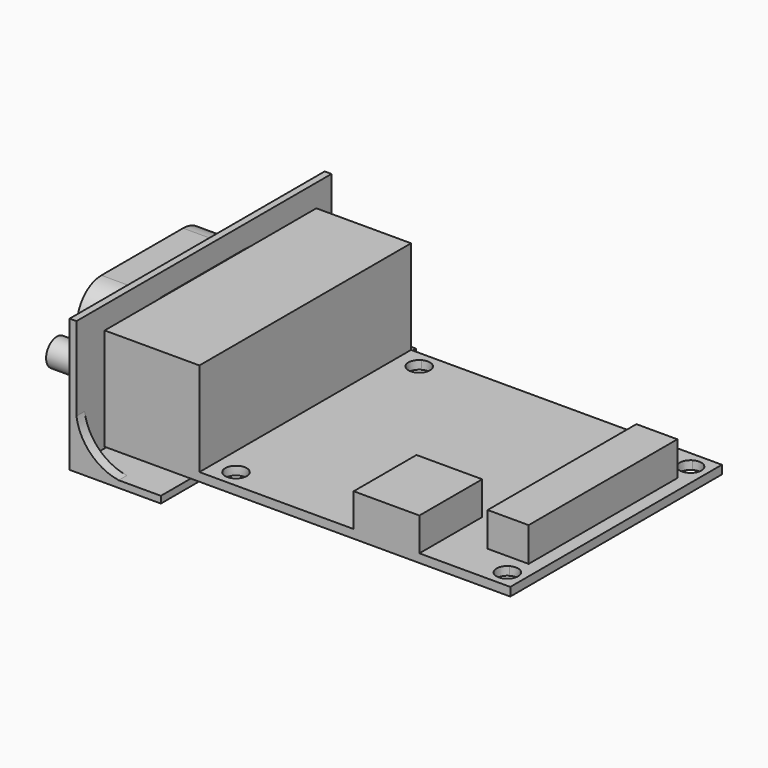
from build123d import *

# Parameters (mm, degrees)
F0_W           = 47.5266514695
F0_H           = 31
F1_DEPTH       = 1
F2_W           = 4.8044053313
F2_H           = 21.7868040781
F3_DEPTH       = 5
F4_W           = 11.1009664834
F4_H           = 31
F5_DEPTH       = 12
F7_R           = 1.5875
F8_DEPTH       = 8
F9_W           = 7.7
F9_H           = 9.2
F10_DEPTH      = 4.9
F11_W          = 55
F11_H          = 37.359307176
F12_DEPTH      = 14
F12_DEPTH_BACK = 1.6
F13_T          = -0.8
F14_OFFSET     = 0.2
F15_W          = 48.7006613985
F15_H          = 51.2911211699
F16_DEPTH      = 25
F18_DEPTH      = 1.2


# Not quite as in the source:
# - ends of sketch curves that miss each other by under 0.0002 mm in the source are joined
# - a pattern or mirror of a feature is missing from the dataset's text; its kind, count and spacing are read off the source's solid


with BuildPart() as f1:
    # F0 (on Top) → F1 (new body)
    with BuildSketch(Plane.XY):
        with Locations((1.27e-05, -1.27e-05)):
            Rectangle(F0_W, F0_H)
        with BuildLine():
            add(Edge.make_bspline(
                [(-13.943801891, -11.7896289619), (-13.943801891, -11.298779652), (-14.205665174, -10.8452147748), (-14.6307564405, -10.5997901198)],
                knots=[0, 0, 0, 0, 1, 1, 1, 1], degree=3))
            add(Edge.make_bspline(
                [(-14.6307564405, -12.9794642726), (-14.205665174, -12.7340396176), (-13.943801891, -12.2804782718), (-13.943801891, -11.7896289619)],
                knots=[0, 0, 0, 0, 1, 1, 1, 1], degree=3))
            add(Edge.make_bspline(
                [(-16.0046620081, -12.9794642726), (-15.5795707416, -13.2248889276), (-15.0558441757, -13.2248889276), (-14.6307564405, -12.9794642726)],
                knots=[0, 0, 0, 0, 1, 1, 1, 1], degree=3))
            add(Edge.make_bspline(
                [(-16.6916130263, -11.7896289619), (-16.6916130263, -12.2804782718), (-16.4297497433, -12.7340396176), (-16.0046620081, -12.9794642726)],
                knots=[0, 0, 0, 0, 1, 1, 1, 1], degree=3))
            add(Edge.make_bspline(
                [(-16.0046620081, -10.5997901198), (-16.4297497433, -10.8452147748), (-16.6916130263, -11.298779652), (-16.6916130263, -11.7896289619)],
                knots=[0, 0, 0, 0, 1, 1, 1, 1], degree=3))
            add(Edge.make_bspline(
                [(-14.6307564405, -10.5997901198), (-15.0558441757, -10.3543654648), (-15.5795707416, -10.3543654648), (-16.0046620081, -10.5997901198)],
                knots=[0, 0, 0, 0, 1, 1, 1, 1], degree=3))
        make_face(mode=Mode.SUBTRACT)
        with BuildLine():
            add(Edge.make_bspline(
                [(-8.7818043126, -13.417529872), (-8.7818043126, -12.7211853521), (-9.3463043262, -12.1566853385), (-10.0426488461, -12.1566853385)],
                knots=[0, 0, 0, 0, 1, 1, 1, 1], degree=3))
            add(Edge.make_bspline(
                [(-9.4122248137, -14.5094538185), (-9.0221190439, -14.2842287237), (-8.7818043126, -13.8679871245), (-8.7818043126, -13.417529872)],
                knots=[0, 0, 0, 0, 1, 1, 1, 1], degree=3))
            add(Edge.make_bspline(
                [(-10.6730728785, -14.5094538185), (-10.2829635774, -14.7346824448), (-9.8023341148, -14.7346824448), (-9.4122248137, -14.5094538185)],
                knots=[0, 0, 0, 0, 1, 1, 1, 1], degree=3))
            add(Edge.make_bspline(
                [(-11.3034933795, -13.417529872), (-11.3034933795, -13.8679871245), (-11.0631786482, -14.2842287237), (-10.6730728785, -14.5094538185)],
                knots=[0, 0, 0, 0, 1, 1, 1, 1], degree=3))
            add(Edge.make_bspline(
                [(-10.0426488461, -12.1566853385), (-10.7389933659, -12.1566853385), (-11.3034933795, -12.7211853521), (-11.3034933795, -13.417529872)],
                knots=[0, 0, 0, 0, 1, 1, 1, 1], degree=3))
        make_face(mode=Mode.SUBTRACT)
        with BuildLine():
            add(Edge.make_bspline(
                [(23.0153119985, -13.4241830138), (23.0153119985, -12.9737257612), (22.7749937359, -12.5574841621), (22.3848879661, -12.3322555358)],
                knots=[0, 0, 0, 0, 1, 1, 1, 1], degree=3))
            add(Edge.make_bspline(
                [(22.3848879661, -14.5161069604), (22.7749937359, -14.2908783341), (23.0153119985, -13.8746367349), (23.0153119985, -13.4241830138)],
                knots=[0, 0, 0, 0, 1, 1, 1, 1], degree=3))
            add(Edge.make_bspline(
                [(21.1240434327, -14.5161069604), (21.5141492024, -14.7413355866), (21.9947821964, -14.7413355866), (22.3848879661, -14.5161069604)],
                knots=[0, 0, 0, 0, 1, 1, 1, 1], degree=3))
            add(Edge.make_bspline(
                [(20.4936194003, -13.4241830138), (20.4936194003, -13.8746367349), (20.7339341315, -14.2908783341), (21.1240434327, -14.5161069604)],
                knots=[0, 0, 0, 0, 1, 1, 1, 1], degree=3))
            add(Edge.make_bspline(
                [(21.1240434327, -12.3322555358), (20.7339341315, -12.5574841621), (20.4936194003, -12.9737257612), (20.4936194003, -13.4241830138)],
                knots=[0, 0, 0, 0, 1, 1, 1, 1], degree=3))
            add(Edge.make_bspline(
                [(22.3848879661, -12.3322555358), (21.9947821964, -12.1070304409), (21.5141492024, -12.1070304409), (21.1240434327, -12.3322555358)],
                knots=[0, 0, 0, 0, 1, 1, 1, 1], degree=3))
        make_face(mode=Mode.SUBTRACT)
        with BuildLine():
            add(Edge.make_bspline(
                [(-14.6307564405, 12.9794353412), (-14.205665174, 12.7340106862), (-13.943801891, 12.2804493404), (-13.943801891, 11.7896000305)],
                knots=[0, 0, 0, 0, 1, 1, 1, 1], degree=3))
            add(Edge.make_bspline(
                [(-13.943801891, 11.7896000305), (-13.943801891, 11.2987507206), (-14.205665174, 10.8451858434), (-14.6307564405, 10.5997611884)],
                knots=[0, 0, 0, 0, 1, 1, 1, 1], degree=3))
            add(Edge.make_bspline(
                [(-14.6307564405, 10.5997611884), (-15.0558441757, 10.3543365334), (-15.5795707416, 10.3543365334), (-16.0046620081, 10.5997611884)],
                knots=[0, 0, 0, 0, 1, 1, 1, 1], degree=3))
            add(Edge.make_bspline(
                [(-16.0046620081, 10.5997611884), (-16.4297497433, 10.8451858434), (-16.6916130263, 11.2987507206), (-16.6916130263, 11.7896000305)],
                knots=[0, 0, 0, 0, 1, 1, 1, 1], degree=3))
            add(Edge.make_bspline(
                [(-16.6916130263, 11.7896000305), (-16.6916130263, 12.2804493404), (-16.4297497433, 12.7340106862), (-16.0046620081, 12.9794353412)],
                knots=[0, 0, 0, 0, 1, 1, 1, 1], degree=3))
            add(Edge.make_bspline(
                [(-16.0046620081, 12.9794353412), (-15.5795707416, 13.2248599962), (-15.0558441757, 13.2248599962), (-14.6307564405, 12.9794353412)],
                knots=[0, 0, 0, 0, 1, 1, 1, 1], degree=3))
        make_face(mode=Mode.SUBTRACT)
        with BuildLine():
            add(Edge.make_bspline(
                [(-9.4122248137, 14.5094248872), (-9.0221190439, 14.2841962609), (-8.7818043126, 13.8679581931), (-8.7818043126, 13.4175009406)],
                knots=[0, 0, 0, 0, 1, 1, 1, 1], degree=3))
            add(Edge.make_bspline(
                [(-8.7818043126, 13.4175009406), (-8.7818043126, 12.7211564207), (-9.3463043262, 12.1566564071), (-10.0426488461, 12.1566564071)],
                knots=[0, 0, 0, 0, 1, 1, 1, 1], degree=3))
            add(Edge.make_bspline(
                [(-10.0426488461, 12.1566564071), (-10.7389933659, 12.1566564071), (-11.3034933795, 12.7211564207), (-11.3034933795, 13.4175009406)],
                knots=[0, 0, 0, 0, 1, 1, 1, 1], degree=3))
            add(Edge.make_bspline(
                [(-11.3034933795, 13.4175009406), (-11.3034933795, 13.8679581931), (-11.0631786482, 14.2841962609), (-10.6730728785, 14.5094248872)],
                knots=[0, 0, 0, 0, 1, 1, 1, 1], degree=3))
            add(Edge.make_bspline(
                [(-10.6730728785, 14.5094248872), (-10.2829635774, 14.7346535134), (-9.8023341148, 14.7346535134), (-9.4122248137, 14.5094248872)],
                knots=[0, 0, 0, 0, 1, 1, 1, 1], degree=3))
        make_face(mode=Mode.SUBTRACT)
        with BuildLine():
            add(Edge.make_bspline(
                [(22.3848879661, 14.516078029), (22.7749937359, 14.2908494027), (23.0153119985, 13.8746078036), (23.0153119985, 13.424150551)],
                knots=[0, 0, 0, 0, 1, 1, 1, 1], degree=3))
            add(Edge.make_bspline(
                [(23.0153119985, 13.424150551), (23.0153119985, 12.9736968298), (22.7749937359, 12.5574552307), (22.3848879661, 12.3322266044)],
                knots=[0, 0, 0, 0, 1, 1, 1, 1], degree=3))
            add(Edge.make_bspline(
                [(22.3848879661, 12.3322266044), (21.9947821964, 12.1069979781), (21.5141492024, 12.1069979781), (21.1240434327, 12.3322266044)],
                knots=[0, 0, 0, 0, 1, 1, 1, 1], degree=3))
            add(Edge.make_bspline(
                [(21.1240434327, 12.3322266044), (20.7339341315, 12.5574552307), (20.4936194003, 12.9736968298), (20.4936194003, 13.424150551)],
                knots=[0, 0, 0, 0, 1, 1, 1, 1], degree=3))
            add(Edge.make_bspline(
                [(20.4936194003, 13.424150551), (20.4936194003, 13.8746078036), (20.7339341315, 14.2908494027), (21.1240434327, 14.516078029)],
                knots=[0, 0, 0, 0, 1, 1, 1, 1], degree=3))
            add(Edge.make_bspline(
                [(21.1240434327, 14.516078029), (21.5141492024, 14.7413066552), (21.9947821964, 14.7413066552), (22.3848879661, 14.516078029)],
                knots=[0, 0, 0, 0, 1, 1, 1, 1], degree=3))
        make_face(mode=Mode.SUBTRACT)
    extrude(amount=F1_DEPTH)

    # F2 (on Top) → F3 (join)
    with BuildSketch(Plane.XY):
        with Locations((19.8277348989, 1.90825e-05)):
            Rectangle(F2_W, F2_H)
    extrude(amount=F3_DEPTH)

    # F4 (on Top) → F5 (join)
    with BuildSketch(Plane.XY):
        with Locations((-18.2128297931, -1.27e-05)):
            Rectangle(F4_W, F4_H)
    extrude(amount=F5_DEPTH)

    # F7 (on offset) → F8 (join)
    with BuildSketch(Plane(origin=(-23.7633130348, 0, 0), x_dir=(0, -1, 0), z_dir=(-1, 0, 0))):
        with Locations((-12.4968001619, 5.9569873847)):
            Circle(F7_R)
        with BuildLine():
            Line((8.8735406381, 3.6322015847), (9.4761048381, 7.0494413847))
            ThreePointArc((9.4761048381, 7.0494413847), (8.6998346843, 9.9464561177), (5.9816236381, 11.2139745847))
            Line((5.9816236381, 11.2139745847), (-5.9816239619, 11.2139745847))
            ThreePointArc((-5.9816239619, 11.2139745847), (-8.6998350081, 9.9464561177), (-9.476099195, 7.0494424368))
            Line((-9.476099195, 7.0494424368), (-8.8735409619, 3.6322015847))
            ThreePointArc((-8.8735409619, 3.6322015847), (-7.6599450056, 1.530142321), (-5.3790851619, 0.6999747847))
            Line((-5.3790851619, 0.6999747847), (5.3790848381, 0.6999747847))
            ThreePointArc((5.3790848381, 0.6999747847), (7.6599446818, 1.530142321), (8.8735406381, 3.6322015847))
        make_face()
        with Locations((12.4967998381, 5.9569873847)):
            Circle(F7_R)
    extrude(amount=F8_DEPTH)

    # F9 (on Top) → F10 (join)
    with BuildSketch(Plane.XY):
        with Locations((9.2633384348, -10.9000127)):
            Rectangle(F9_W, F9_H)
    extrude(amount=F10_DEPTH)


with BuildPart() as f12:
    # F11 (on Top) → F12 (new body, two sides)
    with BuildSketch(Plane.XY) as f12_sk:
        with Locations((2.1668501538, -1.27e-05)):
            Rectangle(F11_W, F11_H)
    extrude(amount=F12_DEPTH)
    extrude(f12_sk.sketch, amount=-F12_DEPTH_BACK)

    # F13
    f13_openings = [f12.faces().sort_by_distance(p)[0] for p in [
        (2.16685, -1.3e-05, 14),
        (29.66685, -1.3e-05, 6.2),
        (2.16685, -18.679666, 6.2),
        (2.16685, 18.679641, 6.2),
    ]]
    offset(amount=F13_T, openings=f13_openings)

    # F14: cut F1, made larger all round first
    f14_tool = offset(f1.part, amount=F14_OFFSET, kind=Kind.INTERSECTION, mode=Mode.PRIVATE)
    add(f14_tool, mode=Mode.SUBTRACT)

    # F15 (on Top) → F16 (cut)
    with BuildSketch(Plane.XY):
        with Locations((9.7142267041, 1.1657075956)):
            Rectangle(F15_W, F15_H)
    extrude(amount=-F16_DEPTH, mode=Mode.SUBTRACT)

    # F17 (on face) → F18 (join)
    with BuildSketch(Plane.XZ.offset(18.679666288)):
        with BuildLine():
            ThreePointArc((-19.5846269207, -0.8), (-22.8781403141, 0.8891826079), (-24.5331498462, 4.2))
            Line((-24.5331498462, 4.2), (-24.5331498462, -0.8))
            Line((-24.5331498462, -0.8), (-19.5846269207, -0.8))
        make_face()
    f18 = extrude(amount=-F18_DEPTH)

    # F18_copies: F18 across plane
    add(f18.mirror(Plane.ZX))


solid = Compound([f1.part, f12.part])
